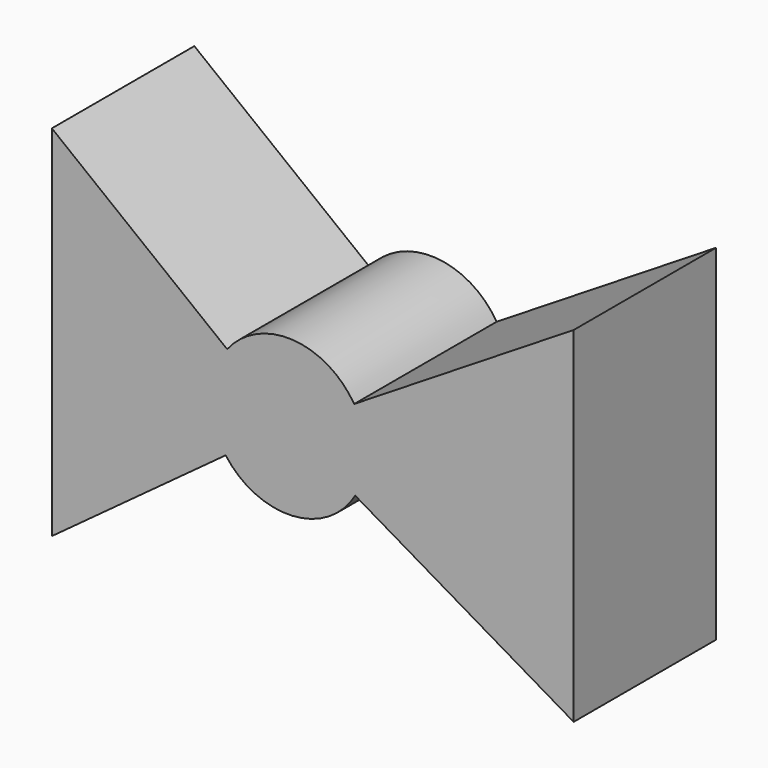
from build123d import *

# Parameters (mm, degrees)
F1_DEPTH = 25.4


with BuildPart() as f1:
    # F0 (on Front) → F1 (new body)
    with BuildSketch(Plane.XZ):
        with BuildLine():
            Line((40.7043881714, -23.8888029385), (40.7043881714, 25.317851454))
            Line((40.7043881714, 25.317851454), (9.4020965094, 5.8480398177))
            ThreePointArc((9.4020965094, 5.8480398177), (10.6466699917, 3.0409548779), (11.0724427513, 0))
            ThreePointArc((11.0724427513, 0), (10.6848861314, -2.9038245196), (9.5493467137, -5.6043702432))
            Line((9.5493467137, -5.6043702432), (40.7043881714, -23.8888029385))
        make_face()
        with BuildLine():
            ThreePointArc((11.0724427513, 0), (10.6466699917, 3.0409548779), (9.4020965094, 5.8480398177))
            Line((9.4020965094, 5.8480398177), (0, 0))
            Line((0, 0), (9.5493467137, -5.6043702432))
            ThreePointArc((9.5493467137, -5.6043702432), (10.6848861314, -2.9038245196), (11.0724427513, 0))
        make_face()
        with BuildLine():
            Line((0, 0), (9.4020965094, 5.8480398177))
            ThreePointArc((9.4020965094, 5.8480398177), (0.6010385922, 11.0561178128), (-8.7127334808, 6.8328078982))
            Line((-8.7127334808, 6.8328078982), (0, 0))
        make_face()
        with BuildLine():
            ThreePointArc((-8.9241617805, -6.5542600647), (0.5685830796, -11.0578344065), (9.5493467137, -5.6043702432))
            Line((9.5493467137, -5.6043702432), (0, 0))
            Line((0, 0), (-8.9241617805, -6.5542600647))
        make_face()
        with BuildLine():
            Line((-8.9241617805, -6.5542600647), (0, 0))
            Line((0, 0), (-8.7127334808, 6.8328078982))
            ThreePointArc((-8.7127334808, 6.8328078982), (-11.0710620889, 0.1748505229), (-8.9241617805, -6.5542600647))
        make_face()
        with BuildLine():
            ThreePointArc((-8.9241617805, -6.5542600647), (-11.0710620889, 0.1748505229), (-8.7127334808, 6.8328078982))
            Line((-8.7127334808, 6.8328078982), (-33.7105058134, 26.4368709177))
            Line((-33.7105058134, 26.4368709177), (-33.7105058134, -24.7583389282))
            Line((-33.7105058134, -24.7583389282), (-8.9241617805, -6.5542600647))
        make_face()
    extrude(amount=F1_DEPTH)


solid = f1.part
